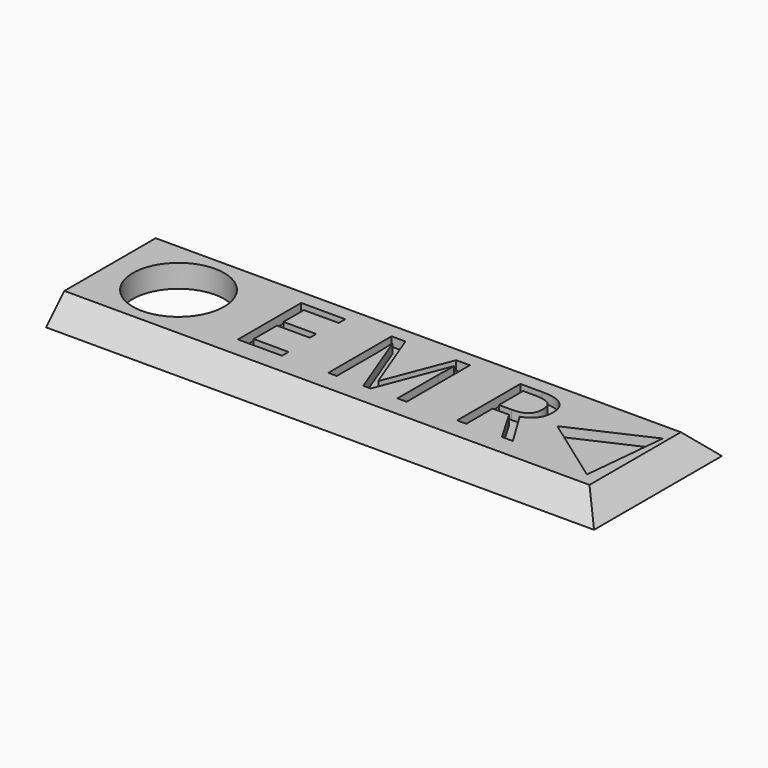
from build123d import *

# Parameters (mm, degrees)
F0_W         = 120
F0_H         = 35
F0_R         = 10
F1_DEPTH     = 5
F2_TEXT_SIZE = 24.2598704062
F3_DEPTH     = 2
F4_SIZE      = 4.99999


# Not quite as in the source:
# - a fillet or chamfer is up to 0.001 mm smaller than in the source, because OpenCascade refuses the exact size
# - Text() gives the source's letters only with a copy of the font that has no kerning and outlines rounded to 1/6400 em; it was checked with that copy


with BuildPart() as f1:
    # F0 (on Top) → F1 (new body)
    with BuildSketch(Plane.XY):
        Rectangle(F0_W, F0_H)
        with Locations((-45, 0)):
            Circle(F0_R, mode=Mode.SUBTRACT)
    extrude(amount=F1_DEPTH)

    # F2 (on face) → F3 (cut)
    with BuildSketch(Plane.XY.offset(5)):
        Polygon((37.1312639619, 1.0390334839), (52.2532872856, -9.7697377205), (54.0529460704, 8.7307042366), align=None)
        with Locations((-27.9769748449, -7.9934215173)):
            Text('E M R', F2_TEXT_SIZE, font='Open Sans', text_align=(TextAlign.LEFT, TextAlign.BOTTOM))
    extrude(amount=-F3_DEPTH, mode=Mode.SUBTRACT)

    # F4 (size 5 in the source; OpenCascade refuses exactly that, so slightly less here)
    f4_edges = [f1.edges().sort_by_distance(p)[0] for p in [
        (0, -17.5, 5),
        (60, 0, 5),
        (0, 17.5, 5),
    ]]
    chamfer(f4_edges, length=F4_SIZE)


solid = f1.part
